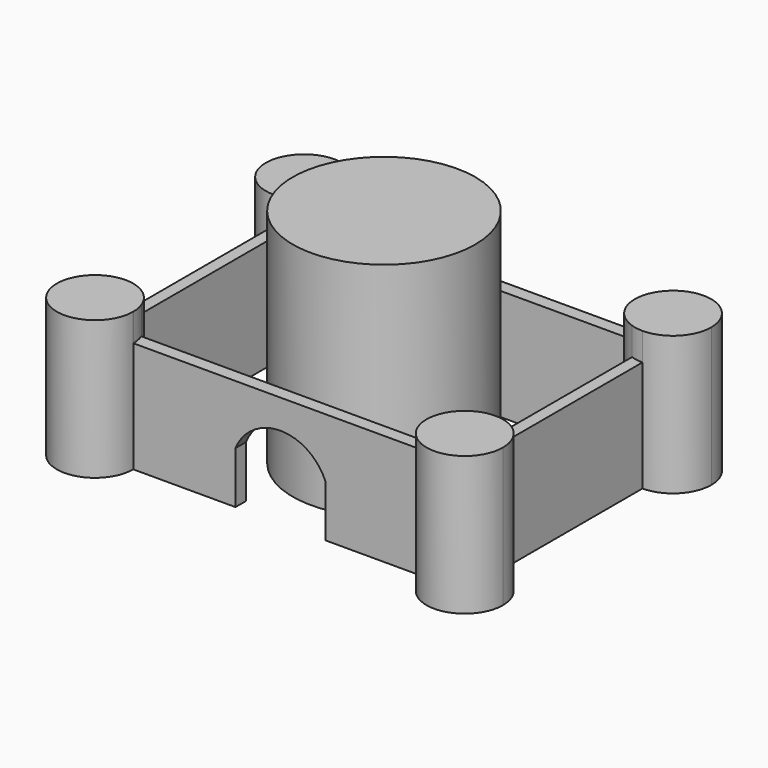
from build123d import *

# Parameters (mm, degrees)
F1_DEPTH = 25.4
F2_DEPTH = 31.75
F0_R     = 20.8784550172
F3_DEPTH = 50.8
F5_DEPTH = 25.4


with BuildPart() as f1:
    # F0 (on Top) → F1 (new body)
    with BuildSketch(Plane.XY):
        with BuildLine():
            ThreePointArc((33.9828109176, 26.9048549235), (33.5914941612, 28.3712616954), (33.4597308818, 29.8832524568))
            Line((33.4597308818, 29.8832524568), (-33.4597346071, 29.8832524568))
            ThreePointArc((-33.4597346071, 29.8832524568), (-33.591497554, 28.3712617257), (-33.9828139678, 26.9048549235))
            Line((-33.9828139678, 26.9048549235), (33.9828109176, 26.9048549235))
        make_face()
    extrude(amount=F1_DEPTH)


with BuildPart() as f1b:
    # F0 (on Top) → F1, piece 2 (new body)
    with BuildSketch(Plane.XY):
        with BuildLine():
            ThreePointArc((-39.4652858377, 21.5813073864), (-40.8155006753, 21.2527209348), (-42.2007255256, 21.1422615383))
            Line((-42.2007255256, 21.1422615383), (-42.2007255256, -21.1567425473))
            ThreePointArc((-42.2007255256, -21.1567425473), (-40.8156954821, -21.2648485586), (-39.4652858377, -21.5910217079))
            Line((-39.4652858377, -21.5910217079), (-39.4652858377, 21.5813073864))
        make_face()
    extrude(amount=F1_DEPTH)


with BuildPart() as f1c:
    # F0 (on Top) → F1, piece 3 (new body)
    with BuildSketch(Plane.XY):
        with BuildLine():
            Line((42.2007255256, -20.9280461702), (42.2007255256, 21.1422634009))
            ThreePointArc((42.2007255256, 21.1422634009), (40.8155007255, 21.2527221915), (39.4652858377, 21.5813080216))
            Line((39.4652858377, 21.5813080216), (39.4652858377, -21.3670920184))
            ThreePointArc((39.4652858377, -21.3670920184), (40.8155006753, -21.0385055668), (42.2007255256, -20.9280461702))
        make_face()
    extrude(amount=F1_DEPTH)


with BuildPart() as f1d:
    # F0 (on Top) → F1, piece 4 (new body)
    with BuildSketch(Plane.XY):
        with BuildLine():
            ThreePointArc((33.4623598882, -29.8832524568), (33.5560958311, -28.3747034059), (33.9083061443, -26.9048549235))
            Line((33.9083061443, -26.9048549235), (-33.9735996091, -26.9048549235))
            ThreePointArc((-33.9735996091, -26.9048549235), (-33.5796202507, -28.3710260767), (-33.4452738296, -29.8832524568))
            Line((-33.4452738296, -29.8832524568), (33.4623598882, -29.8832524568))
        make_face()
    extrude(amount=F1_DEPTH)

    # F4 (on face) → F5 (cut)
    with BuildSketch(Plane.XZ.offset(29.8832524568)):
        with BuildLine():
            Line((-10.068193078, 11.8890367448), (-10.068193078, 0))
            Line((-10.068193078, 0), (10.4966256768, 0))
            Line((10.4966256768, 0), (10.4966256768, 11.8890367448))
            ThreePointArc((10.4966256768, 11.8890367448), (0.2142162994, 18.743975088), (-10.068193078, 11.8890367448))
        make_face()
    extrude(amount=-F5_DEPTH, mode=Mode.SUBTRACT)


with BuildPart() as f2:
    # F0 (on Top) → F2 (new body)
    with BuildSketch(Plane.XY):
        with BuildLine():
            ThreePointArc((-33.9828139678, 26.9048549235), (-33.591497554, 28.3712617257), (-33.4597346071, 29.8832524568))
            ThreePointArc((-33.4597346071, 29.8832524568), (-48.3815394784, 36.0640664096), (-42.2007255256, 21.1422615383))
            ThreePointArc((-42.2007255256, 21.1422615383), (-40.8155006753, 21.2527209348), (-39.4652858377, 21.5813073864))
            ThreePointArc((-39.4652858377, 21.5813073864), (-36.1114714274, 23.6122153205), (-33.9828139678, 26.9048549235))
        make_face()
    extrude(amount=F2_DEPTH)


with BuildPart() as f2b:
    # F0 (on Top) → F2, piece 2 (new body)
    with BuildSketch(Plane.XY):
        with BuildLine():
            ThreePointArc((50.9417127189, 29.8832543194), (42.200720869, 38.624245238), (33.4597308818, 29.8832524568))
            ThreePointArc((33.4597308818, 29.8832524568), (33.5914941612, 28.3712616954), (33.9828109176, 26.9048549235))
            ThreePointArc((33.9828109176, 26.9048549235), (36.1114698198, 23.6122151269), (39.4652858377, 21.5813080216))
            ThreePointArc((39.4652858377, 21.5813080216), (40.8155007255, 21.2527221915), (42.2007255256, 21.1422634009))
            ThreePointArc((42.2007255256, 21.1422634009), (48.3815370702, 23.7024416837), (50.9417127189, 29.8832543194))
        make_face()
    extrude(amount=F2_DEPTH)


with BuildPart() as f2c:
    # F0 (on Top) → F2, piece 3 (new body)
    with BuildSketch(Plane.XY):
        with BuildLine():
            ThreePointArc((50.9417164441, -29.6690370888), (48.3815394784, -23.488223136), (42.2007255256, -20.9280461702))
            ThreePointArc((42.2007255256, -20.9280461702), (40.8155006753, -21.0385055668), (39.4652858377, -21.3670920184))
            ThreePointArc((39.4652858377, -21.3670920184), (36.0306263845, -23.4775268669), (33.9083061443, -26.9048549235))
            ThreePointArc((33.9083061443, -26.9048549235), (33.5560958311, -28.3747034059), (33.4623598882, -29.8832524568))
            ThreePointArc((33.4623598882, -29.8832524568), (42.3078412528, -38.4093716624), (50.9417164441, -29.6690370888))
        make_face()
    extrude(amount=F2_DEPTH)


with BuildPart() as f2d:
    # F0 (on Top) → F2, piece 4 (new body)
    with BuildSketch(Plane.XY):
        with BuildLine():
            ThreePointArc((-39.4652858377, -21.5910217079), (-40.8156954821, -21.2648485586), (-42.2007255256, -21.1567425473))
            ThreePointArc((-42.2007255256, -21.1567425473), (-48.361947715, -36.0836502116), (-33.4452618543, -29.8977214843))
            ThreePointArc((-33.4452618543, -29.8977214843), (-33.4452648481, -29.8904869681), (-33.4452738296, -29.8832524568))
            ThreePointArc((-33.4452738296, -29.8832524568), (-33.5796202507, -28.3710260767), (-33.9735996091, -26.9048549235))
            ThreePointArc((-33.9735996091, -26.9048549235), (-36.1079949651, -23.6160255142), (-39.4652858377, -21.5910217079))
        make_face()
    extrude(amount=F2_DEPTH)


with BuildPart() as f3:
    # F0 (on Top) → F3 (new body)
    with BuildSketch(Plane.XY):
        Circle(F0_R)
    extrude(amount=F3_DEPTH)


solid = Compound([f1.part, f1b.part, f1c.part, f1d.part, f2.part, f2b.part, f2c.part, f2d.part, f3.part])
